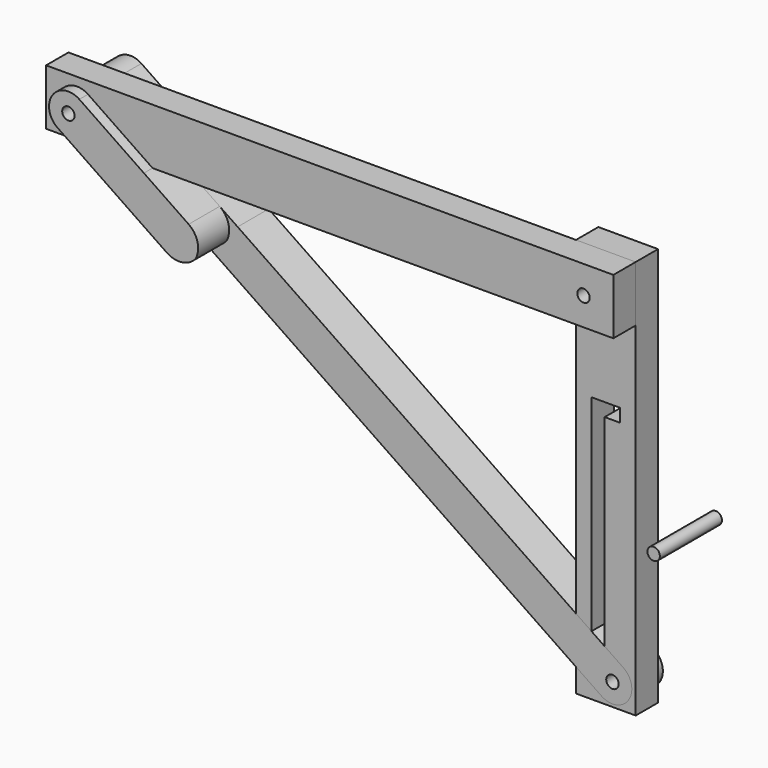
from build123d import *

# Parameters (mm, degrees)
F0_W        = 38.5
F0_H        = 36
F0_R        = 4
F1_DEPTH    = 18
F2_DEPTH    = 18
F3_DEPTH    = 25
F4_R        = 4
F5_DEPTH    = 50
F6_DEPTH    = 25
F7_T1_DEPTH = 95


# Not quite as in the source:
# - a fillet or chamfer that OpenCascade refuses, or shapes differently, is made with other operations: its cross-section is extruded or revolved along the edge and cut away or added


with BuildPart() as f1:
    # F0 (on Front) → F1 (new body)
    with BuildSketch(Plane.XZ):
        with Locations((-19.9438821999, 63.8240744194)):
            Rectangle(F0_W, F0_H)
        with Locations((-19.9438821999, 63.8240744194)):
            Circle(F0_R, mode=Mode.SUBTRACT)
        with BuildLine():
            Line((-0.6938821999, 45.8240744194), (-39.1938821999, 45.8240744194))
            Line((-39.1938821999, 45.8240744194), (-39.1938821999, -130.1749886339))
            Line((-39.1938821999, -130.1749886339), (-29.1938821999, -136.9837487019))
            Line((-29.1938821999, -136.9837487019), (-29.1938821999, -4.1759255806))
            Line((-29.1938821999, -4.1759255806), (-10.6938821999, -4.1759255806))
            Line((-10.6938821999, -4.1759255806), (-10.6938821999, -12.6759255806))
            Line((-10.6938821999, -12.6759255806), (-20.6938821999, -12.6759255806))
            Line((-20.6938821999, -12.6759255806), (-20.6938821999, -142.7711947596))
            Line((-20.6938821999, -142.7711947596), (-8.658818896, -150.9655806035))
            ThreePointArc((-8.658818896, -150.9655806035), (-5.3615114985, -168.3330146088), (-22.7289455038, -171.6303220062))
            Line((-22.7289455038, -171.6303220062), (-39.1938821999, -160.4197416564))
            Line((-39.1938821999, -160.4197416564), (-39.1938821999, -175.5479513049))
            Line((-39.1938821999, -175.5479513049), (-0.6938821999, -175.5479513049))
            Line((-0.6938821999, -175.5479513049), (-0.6938821999, 45.8240744194))
        make_face()
        with BuildLine():
            Line((-29.1938821999, -136.9837487019), (-39.1938821999, -130.1749886339))
            Line((-39.1938821999, -130.1749886339), (-39.1938821999, -160.4197416564))
            Line((-39.1938821999, -160.4197416564), (-22.7289455038, -171.6303220062))
            ThreePointArc((-22.7289455038, -171.6303220062), (-5.3615114985, -168.3330146088), (-8.658818896, -150.9655806035))
            Line((-8.658818896, -150.9655806035), (-20.6938821999, -142.7711947596))
            Line((-20.6938821999, -142.7711947596), (-20.6938821999, -157.0479513049))
            Line((-20.6938821999, -157.0479513049), (-10.6938821999, -157.0479513049))
            Line((-10.6938821999, -157.0479513049), (-10.6938821999, -165.5479513049))
            Line((-10.6938821999, -165.5479513049), (-29.1938821999, -165.5479513049))
            Line((-29.1938821999, -165.5479513049), (-29.1938821999, -136.9837487019))
        make_face()
    extrude(amount=-F1_DEPTH)


with BuildPart() as f2:
    # F0 (on Front) → F2 (new body)
    with BuildSketch(Plane.XZ):
        with BuildLine():
            Line((-39.1938821999, 45.8240744194), (-39.1938821999, 81.8240744194))
            Line((-39.1938821999, 81.8240744194), (-366.3297446435, 81.8240744194))
            Line((-366.3297446435, 81.8240744194), (-366.3297446435, 45.8240744194))
            Line((-366.3297446435, 45.8240744194), (-342.1033899768, 45.8240744194))
            Line((-342.1033899768, 45.8240744194), (-353.3648079474, 53.491703718))
            ThreePointArc((-353.3648079474, 53.491703718), (-356.6621153449, 70.8591377232), (-339.2946813396, 74.1564451207))
            Line((-339.2946813396, 74.1564451207), (-297.6830363138, 45.8240744194))
            Line((-297.6830363138, 45.8240744194), (-39.1938821999, 45.8240744194))
        make_face()
        with Locations((-19.9438821999, 63.8240744194)):
            Rectangle(F0_W, F0_H)
        with Locations((-19.9438821999, 63.8240744194)):
            Circle(F0_R, mode=Mode.SUBTRACT)
        with BuildLine():
            Line((-342.1033899768, 45.8240744194), (-297.6830363138, 45.8240744194))
            Line((-297.6830363138, 45.8240744194), (-339.2946813396, 74.1564451207))
            ThreePointArc((-339.2946813396, 74.1564451207), (-356.6621153449, 70.8591377232), (-353.3648079474, 53.491703718))
            Line((-353.3648079474, 53.491703718), (-342.1033899768, 45.8240744194))
        make_face()
        with Locations((-346.3297446435, 63.8240744194)):
            Circle(F0_R, mode=Mode.SUBTRACT)
    extrude(amount=F2_DEPTH)


with BuildPart() as f3:
    # F0 (on Front) → F3 (new body)
    with BuildSketch(Plane.XZ):
        with BuildLine():
            Line((-29.1938821999, -136.9837487019), (-39.1938821999, -130.1749886339))
            Line((-39.1938821999, -130.1749886339), (-39.1938821999, -160.4197416564))
            Line((-39.1938821999, -160.4197416564), (-22.7289455038, -171.6303220062))
            ThreePointArc((-22.7289455038, -171.6303220062), (-5.3615114985, -168.3330146088), (-8.658818896, -150.9655806035))
            Line((-8.658818896, -150.9655806035), (-20.6938821999, -142.7711947596))
            Line((-20.6938821999, -142.7711947596), (-20.6938821999, -157.0479513049))
            Line((-20.6938821999, -157.0479513049), (-10.6938821999, -157.0479513049))
            Line((-10.6938821999, -157.0479513049), (-10.6938821999, -165.5479513049))
            Line((-10.6938821999, -165.5479513049), (-29.1938821999, -165.5479513049))
            Line((-29.1938821999, -165.5479513049), (-29.1938821999, -136.9837487019))
        make_face()
        Polygon((-39.1938821999, -160.4197416564), (-39.1938821999, -130.1749886339), (-257.2734515904, 18.3101577365), (-271.3435781981, -2.3545836662), align=None)
        Polygon((-20.6938821999, -142.7711947596), (-29.1938821999, -136.9837487019), (-29.1938821999, -165.5479513049), (-10.6938821999, -165.5479513049), (-10.6938821999, -157.0479513049), (-20.6938821999, -157.0479513049), align=None)
        with Locations((-15.6938821999, -161.2979513049)):
            Circle(F0_R, mode=Mode.SUBTRACT)
        with BuildLine():
            Line((-342.1033899768, 45.8240744194), (-297.6830363138, 45.8240744194))
            Line((-297.6830363138, 45.8240744194), (-339.2946813396, 74.1564451207))
            ThreePointArc((-339.2946813396, 74.1564451207), (-356.6621153449, 70.8591377232), (-353.3648079474, 53.491703718))
            Line((-353.3648079474, 53.491703718), (-342.1033899768, 45.8240744194))
        make_face()
        with Locations((-346.3297446435, 63.8240744194)):
            Circle(F0_R, mode=Mode.SUBTRACT)
        Polygon((-257.2734515904, 18.3101577365), (-297.6830363138, 45.8240744194), (-342.1033899768, 45.8240744194), (-271.3435781981, -2.3545836662), align=None)
    extrude(amount=-F3_DEPTH)


with BuildPart() as f5:
    # F4 (on Front) → F5 (new body)
    with BuildSketch(Plane.XZ):
        with Locations((50.8726574481, -46.6468930244)):
            Circle(F4_R)
    extrude(amount=F5_DEPTH)


with BuildPart() as f6:
    # F0 (on Front) → F6 (new body)
    with BuildSketch(Plane.XZ):
        Polygon((-257.2734515904, 18.3101577365), (-297.6830363138, 45.8240744194), (-342.1033899768, 45.8240744194), (-271.3435781981, -2.3545836662), align=None)
        with BuildLine():
            Line((-342.1033899768, 45.8240744194), (-297.6830363138, 45.8240744194))
            Line((-297.6830363138, 45.8240744194), (-339.2946813396, 74.1564451207))
            ThreePointArc((-339.2946813396, 74.1564451207), (-356.6621153449, 70.8591377232), (-353.3648079474, 53.491703718))
            Line((-353.3648079474, 53.491703718), (-342.1033899768, 45.8240744194))
        make_face()
        with Locations((-346.3297446435, 63.8240744194)):
            Circle(F0_R, mode=Mode.SUBTRACT)
    extrude(amount=F6_DEPTH)

    # F7: fillet of radius 14 on 2 edges, made by hand

    # F7_s2 → F7_t1 (cut)
    with BuildSketch(Plane.XZ.offset(-35)):
        with BuildLine():
            ThreePointArc((-265.1527224907, 6.737902551), (-262.9706716765, 17.2285076822), (-268.8457067759, 26.1894286369))
            Line((-268.8457067759, 26.1894286369), (-257.2734515904, 18.3101577365))
            Line((-257.2734515904, 18.3101577365), (-265.1527224907, 6.737902551))
        make_face()
        with BuildLine():
            ThreePointArc((-263.4643072978, 9.2176715193), (-272.4252282525, 3.3426364199), (-282.9158333837, 5.5246872342))
            Line((-282.9158333837, 5.5246872342), (-271.3435781981, -2.3545836662))
            Line((-271.3435781981, -2.3545836662), (-263.4643072978, 9.2176715193))
        make_face()
    extrude(amount=F7_T1_DEPTH, mode=Mode.SUBTRACT)


solid = Compound([f1.part, f2.part, f3.part, f5.part, f6.part])
